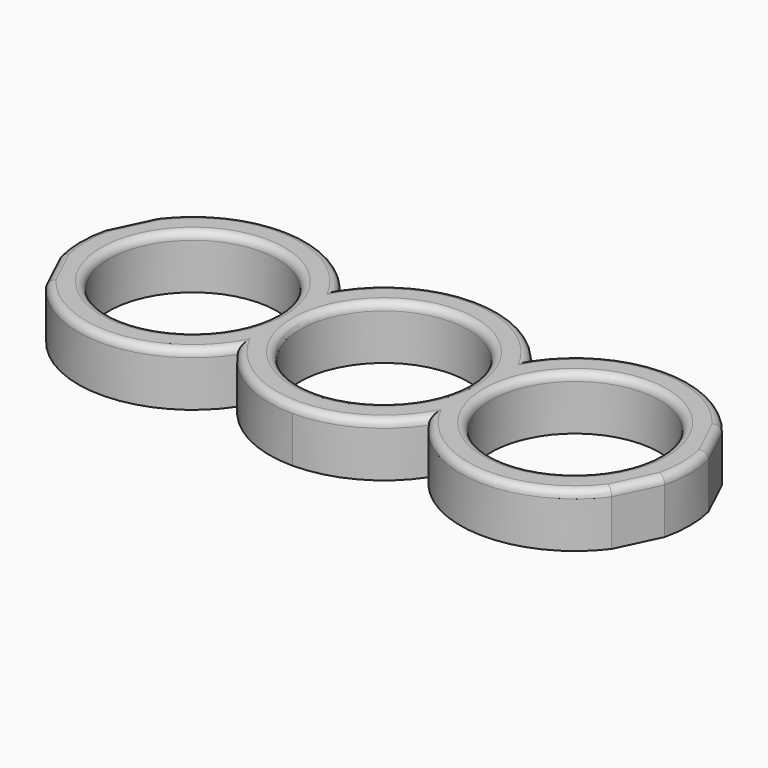
from build123d import *

# Parameters (mm, degrees)
F0_R          = 11
F1_DEPTH      = 7
F2_T1_DEPTH   = 14.5299562036
F2_T3_DEPTH   = 14.5299562036
F2_T5_DEPTH   = 14.5299562036
F2_T7_DEPTH   = 14.5299562036
F2_T12_ANGLE  = 46.6991172175
F2_T16_ANGLE  = 128.5620164001
F2_S17_R      = 15
F2_T18_DEPTH  = 17
F2_T22_ANGLE  = 131.9960454578
F2_S23_R      = 15
F2_T24_DEPTH  = 17
F2_S25_R      = 15
F2_T26_DEPTH  = 17
F2_T30_ANGLE  = 128.5620164001
F2_S31_R      = 15
F2_T32_DEPTH  = 17
F2_T34_ANGLE  = 46.6991172175
F2_T38_ANGLE  = 128.5620164001
F2_S39_R      = 15
F2_T40_DEPTH  = 17
F2_T44_ANGLE  = 131.9960454578
F2_S45_R      = 15
F2_T46_DEPTH  = 17
F2_S47_R      = 15
F2_T48_DEPTH  = 17
F2_T52_ANGLE  = 128.5620164001
F2_S53_R      = 15
F2_T54_DEPTH  = 17
F2_T63_ANGLE  = 128.5620164001
F2_S64_R      = 15
F2_T65_DEPTH  = 17
F2_T68_ANGLE  = 131.9960454578
F2_S69_R      = 15
F2_T70_DEPTH  = 17
F2_T76_ANGLE  = 131.9960454578
F2_S77_R      = 15
F2_T78_DEPTH  = 17
F2_T81_ANGLE  = 128.5620164001
F2_S82_R      = 15
F2_T83_DEPTH  = 17
F2_T89_ANGLE  = 128.5620164001
F2_S90_R      = 15
F2_T91_DEPTH  = 17
F2_T94_ANGLE  = 131.9960454578
F2_S95_R      = 15
F2_T96_DEPTH  = 17
F2_T102_ANGLE = 131.9960454578
F2_S103_R     = 15
F2_T104_DEPTH = 17
F2_T107_ANGLE = 128.5620164001
F2_S108_R     = 15
F2_T109_DEPTH = 17


# Not quite as in the source:
# - a fillet or chamfer that OpenCascade refuses, or shapes differently, is made with other operations: its cross-section is extruded or revolved along the edge and cut away or added


with BuildPart() as f1:
    # F0 (on Top) → F1 (new body)
    with BuildSketch(Plane.XY):
        with BuildLine():
            ThreePointArc((-36.9810110821, -9.0252630682), (-24.5506485813, -14.9932679327), (-12.5, -8.2915619759))
            ThreePointArc((-12.5, -8.2915619759), (-7.0931858273, -13.2169101843), (0, -15))
            ThreePointArc((0, -15), (7.0931858273, -13.2169101843), (12.5, -8.2915619759))
            ThreePointArc((12.5, -8.2915619759), (24.5506485813, -14.9932679327), (36.9810110821, -9.0252630682))
            add(Edge.make_bspline(
                [(39.5670203583, -3.577976786), (38.7050172662, -5.39373888), (37.8430141742, -7.2095009741), (36.9810110821, -9.0252630682)],
                knots=[0, 0, 0, 0, 6.0299562036, 6.0299562036, 6.0299562036, 6.0299562036], degree=3))
            ThreePointArc((39.5670203583, -3.577976786), (40, 0), (39.5670203583, 3.577976786))
            add(Edge.make_bspline(
                [(36.9810110821, 9.0252630682), (37.8430141742, 7.2095009741), (38.7050172662, 5.39373888), (39.5670203583, 3.577976786)],
                knots=[0, 0, 0, 0, 6.0299562036, 6.0299562036, 6.0299562036, 6.0299562036], degree=3))
            ThreePointArc((36.9810110821, 9.0252630682), (24.5506485813, 14.9932679327), (12.5, 8.2915619759))
            ThreePointArc((12.5, 8.2915619759), (7.0931858273, 13.2169101843), (0, 15))
            ThreePointArc((0, 15), (-7.0931858273, 13.2169101843), (-12.5, 8.2915619759))
            ThreePointArc((-12.5, 8.2915619759), (-24.5506485813, 14.9932679327), (-36.9810110821, 9.0252630682))
            add(Edge.make_bspline(
                [(-36.9810110821, 9.0252630682), (-37.8430141742, 7.2095009741), (-38.7050172662, 5.39373888), (-39.5670203583, 3.577976786)],
                knots=[0, 0, 0, 0, 6.0299562036, 6.0299562036, 6.0299562036, 6.0299562036], degree=3))
            ThreePointArc((-39.5670203583, 3.577976786), (-40, 0), (-39.5670203583, -3.577976786))
            add(Edge.make_bspline(
                [(-39.5670203583, -3.577976786), (-38.7050172662, -5.39373888), (-37.8430141742, -7.2095009741), (-36.9810110821, -9.0252630682)],
                knots=[0, 0, 0, 0, 6.0299562036, 6.0299562036, 6.0299562036, 6.0299562036], degree=3))
        make_face()
        with Locations((-25, 0)):
            Circle(F0_R, mode=Mode.SUBTRACT)
        with BuildLine():
            ThreePointArc((0, -11), (-11, 0), (0, 11))
            ThreePointArc((0, 11), (11, 0), (0, -11))
        make_face(mode=Mode.SUBTRACT)
        with Locations((25, 0)):
            Circle(F0_R, mode=Mode.SUBTRACT)
    extrude(amount=F1_DEPTH)

    # F2: fillet of radius 1 on 15 edges, made by hand

    # F2_s2 → F2_t1 (cut)
    with BuildSketch(Plane(origin=(-7.7136917523, 16.2484673409, 0), x_dir=(0, 0, 1), z_dir=(0.4288603746, -0.9033707872, 0))):
        with BuildLine():
            ThreePointArc((7, 36.2781427917), (6.7071067812, 36.9852495729), (6, 37.2781427917))
            Line((6, 37.2781427917), (7, 37.2781427917))
            Line((7, 37.2781427917), (7, 36.2781427917))
        make_face()
    extrude(amount=F2_T1_DEPTH, mode=Mode.SUBTRACT)

    # F2_s4 → F2_t3 (cut)
    with BuildSketch(Plane(origin=(7.7136917523, 16.2484673409, 0), x_dir=(0, 0, 1), z_dir=(-0.4288603746, -0.9033707872, 0))):
        with BuildLine():
            ThreePointArc((7, -36.2781427917), (6.7071067812, -36.9852495729), (6, -37.2781427917))
            Line((6, -37.2781427917), (7, -37.2781427917))
            Line((7, -37.2781427917), (7, -36.2781427917))
        make_face()
    extrude(amount=F2_T3_DEPTH, mode=Mode.SUBTRACT)

    # F2_s6 → F2_t5 (cut)
    with BuildSketch(Plane(origin=(1.4823692921, -3.1225293677, 0), x_dir=(0, 0, 1), z_dir=(0.4288603746, -0.9033707872, 0))):
        with BuildLine():
            ThreePointArc((7, -36.2781427917), (6.7071067812, -36.9852495729), (6, -37.2781427917))
            Line((6, -37.2781427917), (7, -37.2781427917))
            Line((7, -37.2781427917), (7, -36.2781427917))
        make_face()
    extrude(amount=F2_T5_DEPTH, mode=Mode.SUBTRACT)

    # F2_s8 → F2_t7 (cut)
    with BuildSketch(Plane(origin=(-1.4823692921, -3.1225293677, 0), x_dir=(0, 0, 1), z_dir=(-0.4288603746, -0.9033707872, 0))):
        with BuildLine():
            ThreePointArc((7, 36.2781427917), (6.7071067812, 36.9852495729), (6, 37.2781427917))
            Line((6, 37.2781427917), (7, 37.2781427917))
            Line((7, 37.2781427917), (7, 36.2781427917))
        make_face()
    extrude(amount=F2_T7_DEPTH, mode=Mode.SUBTRACT)

    # F2_s9 → F2_t10 (revolve, cut)
    with BuildSketch(Plane.XZ):
        with BuildLine():
            ThreePointArc((-13, 7), (-13.7071067812, 6.7071067812), (-14, 6))
            Line((-14, 6), (-14, 7))
            Line((-14, 7), (-13, 7))
        make_face()
    revolve(axis=Axis((-25, 0, 7), (0, 0, 1)), mode=Mode.SUBTRACT)

    # F2_s11 → F2_t12 (revolve, cut)
    with BuildSketch(Plane(origin=(-3.9271304253, -9.0970273856, 0), x_dir=(0, 0, 1), z_dir=(0.3963397747, 0.9181039064, 0))):
        with BuildLine():
            ThreePointArc((6, -37.9525976606), (6.7071067812, -37.6597044417), (7, -36.9525976606))
            Line((7, -36.9525976606), (7, -37.9525976606))
            Line((7, -37.9525976606), (6, -37.9525976606))
        make_face()
    revolve(axis=Axis((-25, 0, 7), (0, 0, 1)), revolution_arc=F2_T12_ANGLE, mode=Mode.SUBTRACT)


with BuildPart() as f2_tool14:
    # F2_s15 → F2_t16 (revolve)
    with BuildSketch(Plane(origin=(-5.3073105904, 10.2232685114, 0), x_dir=(0, 0, 1), z_dir=(-0.4607520197, 0.8875289158, 0))):
        with BuildLine():
            ThreePointArc((7, -36.188222895), (6.7071067812, -36.8953296762), (6, -37.188222895))
            Line((6, -37.188222895), (7, -37.188222895))
            Line((7, -37.188222895), (7, -36.188222895))
        make_face()
    revolve(axis=Axis((-25, 0, 7), (0, 0, 1)), revolution_arc=F2_T16_ANGLE)

    # F2_s17 → F2_t18 (cut, symmetric)
    with BuildSketch(Plane.XY.offset(6.1)):
        Circle(F2_S17_R)
    extrude(amount=F2_T18_DEPTH, both=True, mode=Mode.SUBTRACT)


with BuildPart() as f1_1:
    add(f1.part)

    # F2_t13: cut F2_tool14
    add(f2_tool14.part, mode=Mode.SUBTRACT)


with BuildPart() as f2_tool20:
    # F2_s21 → F2_t22 (revolve)
    with BuildSketch(Plane(origin=(0, 0, 0), x_dir=(0, 0, 1), z_dir=(0.4067681692, 0.9135314207, 0))):
        with BuildLine():
            ThreePointArc((7, 14), (6.7071067812, 14.7071067812), (6, 15))
            Line((6, 15), (7, 15))
            Line((7, 15), (7, 14))
        make_face()
    revolve(axis=Axis((0, 0, 7), (0, 0, -1)), revolution_arc=F2_T22_ANGLE)

    # F2_s23 → F2_t24 (cut, symmetric)
    with BuildSketch(Plane.XY.offset(6.1)):
        with Locations((25, 0)):
            Circle(F2_S23_R)
    extrude(amount=F2_T24_DEPTH, both=True, mode=Mode.SUBTRACT)

    # F2_s25 → F2_t26 (cut, symmetric)
    with BuildSketch(Plane.XY.offset(6.1)):
        with Locations((-25, 0)):
            Circle(F2_S25_R)
    extrude(amount=F2_T26_DEPTH, both=True, mode=Mode.SUBTRACT)


with BuildPart() as f1_2:
    add(f1_1.part)

    # F2_t19: cut F2_tool20
    add(f2_tool20.part, mode=Mode.SUBTRACT)


with BuildPart() as f2_tool28:
    # F2_s29 → F2_t30 (revolve)
    with BuildSketch(Plane(origin=(4.1366258853, -9.2899931871, 0), x_dir=(0, 0, 1), z_dir=(-0.4067739365, 0.9135288526, 0))):
        with BuildLine():
            ThreePointArc((7, 8.8382213158), (6.7071067812, 8.1311145346), (6, 7.8382213158))
            Line((6, 7.8382213158), (7, 7.8382213158))
            Line((7, 7.8382213158), (7, 8.8382213158))
        make_face()
    revolve(axis=Axis((25, 0, 7), (0, 0, 1)), revolution_arc=F2_T30_ANGLE)

    # F2_s31 → F2_t32 (cut, symmetric)
    with BuildSketch(Plane.XY.offset(6.1)):
        Circle(F2_S31_R)
    extrude(amount=F2_T32_DEPTH, both=True, mode=Mode.SUBTRACT)


with BuildPart() as f1_3:
    add(f1_2.part)

    # F2_t27: cut F2_tool28
    add(f2_tool28.part, mode=Mode.SUBTRACT)

    # F2_s33 → F2_t34 (revolve, cut)
    with BuildSketch(Plane(origin=(3.9271304253, 9.0970273856, 0), x_dir=(0, 0, 1), z_dir=(-0.3963397747, -0.9181039064, 0))):
        with BuildLine():
            ThreePointArc((7, -36.9525976606), (6.7071067812, -37.6597044417), (6, -37.9525976606))
            Line((6, -37.9525976606), (7, -37.9525976606))
            Line((7, -37.9525976606), (7, -36.9525976606))
        make_face()
    revolve(axis=Axis((25, 0, 7), (0, 0, 1)), revolution_arc=F2_T34_ANGLE, mode=Mode.SUBTRACT)


with BuildPart() as f2_tool36:
    # F2_s37 → F2_t38 (revolve)
    with BuildSketch(Plane(origin=(5.3073105904, -10.2232685114, 0), x_dir=(0, 0, 1), z_dir=(0.4607520197, -0.8875289158, 0))):
        with BuildLine():
            ThreePointArc((7, -36.188222895), (6.7071067812, -36.8953296762), (6, -37.188222895))
            Line((6, -37.188222895), (7, -37.188222895))
            Line((7, -37.188222895), (7, -36.188222895))
        make_face()
    revolve(axis=Axis((25, 0, 7), (0, 0, 1)), revolution_arc=F2_T38_ANGLE)

    # F2_s39 → F2_t40 (cut, symmetric)
    with BuildSketch(Plane.XY.offset(6.1)):
        Circle(F2_S39_R)
    extrude(amount=F2_T40_DEPTH, both=True, mode=Mode.SUBTRACT)


with BuildPart() as f1_4:
    add(f1_3.part)

    # F2_t35: cut F2_tool36
    add(f2_tool36.part, mode=Mode.SUBTRACT)


with BuildPart() as f2_tool42:
    # F2_s43 → F2_t44 (revolve)
    with BuildSketch(Plane(origin=(0, 0, 0), x_dir=(0, 0, 1), z_dir=(-0.4067681692, -0.9135314207, 0))):
        with BuildLine():
            ThreePointArc((7, 14), (6.7071067812, 14.7071067812), (6, 15))
            Line((6, 15), (7, 15))
            Line((7, 15), (7, 14))
        make_face()
    revolve(axis=Axis((0, 0, 7), (0, 0, -1)), revolution_arc=F2_T44_ANGLE)

    # F2_s45 → F2_t46 (cut, symmetric)
    with BuildSketch(Plane.XY.offset(6.1)):
        with Locations((-25, 0)):
            Circle(F2_S45_R)
    extrude(amount=F2_T46_DEPTH, both=True, mode=Mode.SUBTRACT)

    # F2_s47 → F2_t48 (cut, symmetric)
    with BuildSketch(Plane.XY.offset(6.1)):
        with Locations((25, 0)):
            Circle(F2_S47_R)
    extrude(amount=F2_T48_DEPTH, both=True, mode=Mode.SUBTRACT)


with BuildPart() as f1_5:
    add(f1_4.part)

    # F2_t41: cut F2_tool42
    add(f2_tool42.part, mode=Mode.SUBTRACT)


with BuildPart() as f2_tool50:
    # F2_s51 → F2_t52 (revolve)
    with BuildSketch(Plane(origin=(-4.1366258853, 9.2899931871, 0), x_dir=(0, 0, 1), z_dir=(0.4067739365, -0.9135288526, 0))):
        with BuildLine():
            ThreePointArc((7, 8.8382213158), (6.7071067812, 8.1311145346), (6, 7.8382213158))
            Line((6, 7.8382213158), (7, 7.8382213158))
            Line((7, 7.8382213158), (7, 8.8382213158))
        make_face()
    revolve(axis=Axis((-25, 0, 7), (0, 0, 1)), revolution_arc=F2_T52_ANGLE)

    # F2_s53 → F2_t54 (cut, symmetric)
    with BuildSketch(Plane.XY.offset(6.1)):
        Circle(F2_S53_R)
    extrude(amount=F2_T54_DEPTH, both=True, mode=Mode.SUBTRACT)


with BuildPart() as f1_6:
    add(f1_5.part)

    # F2_t49: cut F2_tool50
    add(f2_tool50.part, mode=Mode.SUBTRACT)

    # F2_s55 → F2_t56 (revolve, cut)
    with BuildSketch(Plane.YZ):
        with BuildLine():
            ThreePointArc((-12, 7), (-11.2928932188, 6.7071067812), (-11, 6))
            Line((-11, 6), (-11, 7))
            Line((-11, 7), (-12, 7))
        make_face()
    revolve(axis=Axis((0, 0, 7), (0, 0, 1)), mode=Mode.SUBTRACT)

    # F2_s57 → F2_t58 (revolve, cut)
    with BuildSketch(Plane.XZ):
        with BuildLine():
            ThreePointArc((37, 7), (36.2928932188, 6.7071067812), (36, 6))
            Line((36, 6), (36, 7))
            Line((36, 7), (37, 7))
        make_face()
    revolve(axis=Axis((25, 0, 7), (0, 0, 1)), mode=Mode.SUBTRACT)


with BuildPart() as f2_tool61:
    # F2_s62 → F2_t63 (revolve)
    with BuildSketch(Plane(origin=(-5.3073105904, 10.2232685114, 0), x_dir=(0, 0, 1), z_dir=(-0.4607520197, 0.8875289158, 0))):
        with BuildLine():
            ThreePointArc((7, -36.188222895), (6.7071067812, -36.8953296762), (6, -37.188222895))
            Line((6, -37.188222895), (7, -37.188222895))
            Line((7, -37.188222895), (7, -36.188222895))
        make_face()
    revolve(axis=Axis((-25, 0, 7), (0, 0, 1)), revolution_arc=F2_T63_ANGLE)

    # F2_s64 → F2_t65 (intersect, symmetric)
    with BuildSketch(Plane.XY.offset(6.1)):
        Circle(F2_S64_R)
    extrude(amount=F2_T65_DEPTH, both=True, mode=Mode.INTERSECT)


with BuildPart() as f2_tool66:
    # F2_s67 → F2_t68 (revolve)
    with BuildSketch(Plane(origin=(0, 0, 0), x_dir=(0, 0, 1), z_dir=(0.4067681692, 0.9135314207, 0))):
        with BuildLine():
            ThreePointArc((7, 14), (6.7071067812, 14.7071067812), (6, 15))
            Line((6, 15), (7, 15))
            Line((7, 15), (7, 14))
        make_face()
    revolve(axis=Axis((0, 0, 7), (0, 0, -1)), revolution_arc=F2_T68_ANGLE)

    # F2_s69 → F2_t70 (intersect, symmetric)
    with BuildSketch(Plane.XY.offset(6.1)):
        with Locations((-25, 0)):
            Circle(F2_S69_R)
    extrude(amount=F2_T70_DEPTH, both=True, mode=Mode.INTERSECT)


with BuildPart() as f2_tool61_1:
    add(f2_tool61.part)

    # F2_t71: intersect F2_tool66
    add(f2_tool66.part, mode=Mode.INTERSECT)


with BuildPart() as f1_7:
    add(f1_6.part)

    # F2_t59: cut F2_tool61
    add(f2_tool61_1.part, mode=Mode.SUBTRACT)


with BuildPart() as f2_tool74:
    # F2_s75 → F2_t76 (revolve)
    with BuildSketch(Plane(origin=(0, 0, 0), x_dir=(0, 0, 1), z_dir=(0.4067681692, 0.9135314207, 0))):
        with BuildLine():
            ThreePointArc((7, 14), (6.7071067812, 14.7071067812), (6, 15))
            Line((6, 15), (7, 15))
            Line((7, 15), (7, 14))
        make_face()
    revolve(axis=Axis((0, 0, 7), (0, 0, -1)), revolution_arc=F2_T76_ANGLE)

    # F2_s77 → F2_t78 (intersect, symmetric)
    with BuildSketch(Plane.XY.offset(6.1)):
        with Locations((25, 0)):
            Circle(F2_S77_R)
    extrude(amount=F2_T78_DEPTH, both=True, mode=Mode.INTERSECT)


with BuildPart() as f2_tool79:
    # F2_s80 → F2_t81 (revolve)
    with BuildSketch(Plane(origin=(4.1366258853, -9.2899931871, 0), x_dir=(0, 0, 1), z_dir=(-0.4067739365, 0.9135288526, 0))):
        with BuildLine():
            ThreePointArc((7, 8.8382213158), (6.7071067812, 8.1311145346), (6, 7.8382213158))
            Line((6, 7.8382213158), (7, 7.8382213158))
            Line((7, 7.8382213158), (7, 8.8382213158))
        make_face()
    revolve(axis=Axis((25, 0, 7), (0, 0, 1)), revolution_arc=F2_T81_ANGLE)

    # F2_s82 → F2_t83 (intersect, symmetric)
    with BuildSketch(Plane.XY.offset(6.1)):
        Circle(F2_S82_R)
    extrude(amount=F2_T83_DEPTH, both=True, mode=Mode.INTERSECT)


with BuildPart() as f2_tool74_1:
    add(f2_tool74.part)

    # F2_t84: intersect F2_tool79
    add(f2_tool79.part, mode=Mode.INTERSECT)


with BuildPart() as f1_8:
    add(f1_7.part)

    # F2_t72: cut F2_tool74
    add(f2_tool74_1.part, mode=Mode.SUBTRACT)


with BuildPart() as f2_tool87:
    # F2_s88 → F2_t89 (revolve)
    with BuildSketch(Plane(origin=(5.3073105904, -10.2232685114, 0), x_dir=(0, 0, 1), z_dir=(0.4607520197, -0.8875289158, 0))):
        with BuildLine():
            ThreePointArc((7, -36.188222895), (6.7071067812, -36.8953296762), (6, -37.188222895))
            Line((6, -37.188222895), (7, -37.188222895))
            Line((7, -37.188222895), (7, -36.188222895))
        make_face()
    revolve(axis=Axis((25, 0, 7), (0, 0, 1)), revolution_arc=F2_T89_ANGLE)

    # F2_s90 → F2_t91 (intersect, symmetric)
    with BuildSketch(Plane.XY.offset(6.1)):
        Circle(F2_S90_R)
    extrude(amount=F2_T91_DEPTH, both=True, mode=Mode.INTERSECT)


with BuildPart() as f2_tool92:
    # F2_s93 → F2_t94 (revolve)
    with BuildSketch(Plane(origin=(0, 0, 0), x_dir=(0, 0, 1), z_dir=(-0.4067681692, -0.9135314207, 0))):
        with BuildLine():
            ThreePointArc((7, 14), (6.7071067812, 14.7071067812), (6, 15))
            Line((6, 15), (7, 15))
            Line((7, 15), (7, 14))
        make_face()
    revolve(axis=Axis((0, 0, 7), (0, 0, -1)), revolution_arc=F2_T94_ANGLE)

    # F2_s95 → F2_t96 (intersect, symmetric)
    with BuildSketch(Plane.XY.offset(6.1)):
        with Locations((25, 0)):
            Circle(F2_S95_R)
    extrude(amount=F2_T96_DEPTH, both=True, mode=Mode.INTERSECT)


with BuildPart() as f2_tool87_1:
    add(f2_tool87.part)

    # F2_t97: intersect F2_tool92
    add(f2_tool92.part, mode=Mode.INTERSECT)


with BuildPart() as f1_9:
    add(f1_8.part)

    # F2_t85: cut F2_tool87
    add(f2_tool87_1.part, mode=Mode.SUBTRACT)


with BuildPart() as f2_tool100:
    # F2_s101 → F2_t102 (revolve)
    with BuildSketch(Plane(origin=(0, 0, 0), x_dir=(0, 0, 1), z_dir=(-0.4067681692, -0.9135314207, 0))):
        with BuildLine():
            ThreePointArc((7, 14), (6.7071067812, 14.7071067812), (6, 15))
            Line((6, 15), (7, 15))
            Line((7, 15), (7, 14))
        make_face()
    revolve(axis=Axis((0, 0, 7), (0, 0, -1)), revolution_arc=F2_T102_ANGLE)

    # F2_s103 → F2_t104 (intersect, symmetric)
    with BuildSketch(Plane.XY.offset(6.1)):
        with Locations((-25, 0)):
            Circle(F2_S103_R)
    extrude(amount=F2_T104_DEPTH, both=True, mode=Mode.INTERSECT)


with BuildPart() as f2_tool105:
    # F2_s106 → F2_t107 (revolve)
    with BuildSketch(Plane(origin=(-4.1366258853, 9.2899931871, 0), x_dir=(0, 0, 1), z_dir=(0.4067739365, -0.9135288526, 0))):
        with BuildLine():
            ThreePointArc((7, 8.8382213158), (6.7071067812, 8.1311145346), (6, 7.8382213158))
            Line((6, 7.8382213158), (7, 7.8382213158))
            Line((7, 7.8382213158), (7, 8.8382213158))
        make_face()
    revolve(axis=Axis((-25, 0, 7), (0, 0, 1)), revolution_arc=F2_T107_ANGLE)

    # F2_s108 → F2_t109 (intersect, symmetric)
    with BuildSketch(Plane.XY.offset(6.1)):
        Circle(F2_S108_R)
    extrude(amount=F2_T109_DEPTH, both=True, mode=Mode.INTERSECT)


with BuildPart() as f2_tool100_1:
    add(f2_tool100.part)

    # F2_t110: intersect F2_tool105
    add(f2_tool105.part, mode=Mode.INTERSECT)


with BuildPart() as f1_10:
    add(f1_9.part)

    # F2_t98: cut F2_tool100
    add(f2_tool100_1.part, mode=Mode.SUBTRACT)


solid = f1_10.part
